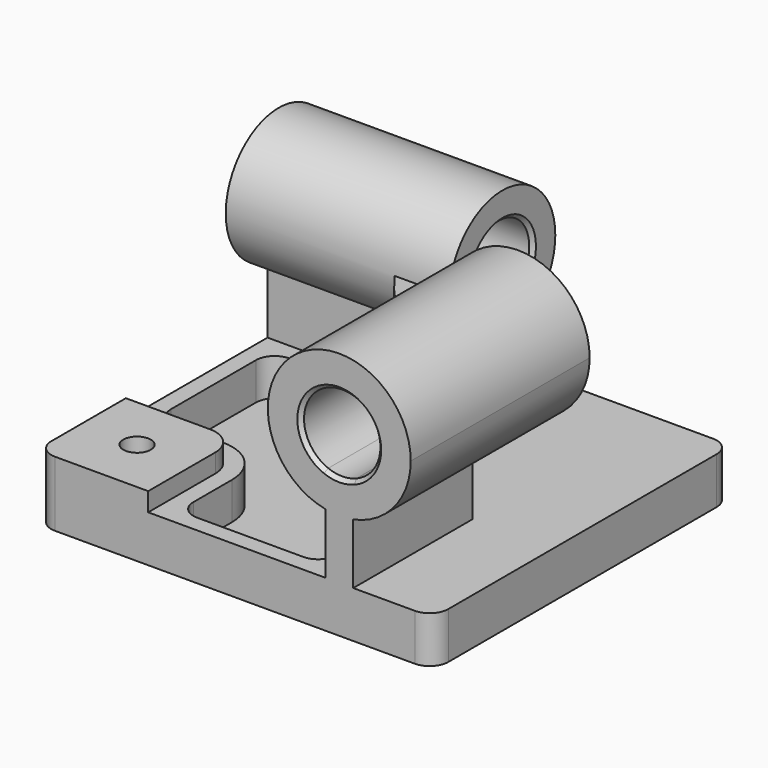
from build123d import *

# Parameters (mm, degrees)
F1_DEPTH       = 35
F2_DEPTH       = 25
F3_DEPTH       = 5
F4_DEPTH       = 95
F5_D           = 14.75
F5_CBORE_D     = 22.25
F5_CBORE_DEPTH = 14
F6_DEPTH       = 25
F8_DEPTH       = 120
F9_DEPTH       = 120
F11_DEPTH      = 120
F12_DEPTH      = 120
F13_SIZE       = 2


with BuildPart() as f1:
    # F0 (on Top) → F1 (new body)
    with BuildSketch(Plane.XY):
        with BuildLine():
            ThreePointArc((-106.5, 10), (-103.5710678119, 2.9289321881), (-96.5, 0))
            Line((-96.5, 0), (-46.5, 0))
            Line((-46.5, 0), (-46.5, 45))
            ThreePointArc((-46.5, 45), (-50.8933982822, 55.6066017178), (-61.5, 60))
            Line((-61.5, 60), (-106.5, 60))
            Line((-106.5, 60), (-106.5, 10))
        make_face()
    extrude(amount=F1_DEPTH)

    # F0 (on Top) → F2 (join)
    with BuildSketch(Plane.XY):
        with BuildLine():
            Line((-46.5, 45), (-46.5, 0))
            Line((-46.5, 0), (48.5, 0))
            Line((48.5, 0), (48.5, 9))
            Line((48.5, 9), (48.5, 73.0645805597))
            ThreePointArc((48.5, 73.0645805597), (0.9989947663, 106.8341893096), (-31.8154327598, 155))
            Line((-31.8154327598, 155), (-106.5, 155))
            Line((-106.5, 155), (-106.5, 60))
            Line((-106.5, 60), (-61.5, 60))
            ThreePointArc((-61.5, 60), (-50.8933982822, 55.6066017178), (-46.5, 45))
        make_face()
        with BuildLine():
            Line((-61.5, 69), (-87.5, 69))
            ThreePointArc((-87.5, 69), (-94.5710678119, 71.9289321881), (-97.5, 79))
            Line((-97.5, 79), (-97.5, 136))
            ThreePointArc((-97.5, 136), (-94.5710678119, 143.0710678119), (-87.5, 146))
            Line((-87.5, 146), (-44.0372922197, 146))
            ThreePointArc((-44.0372922197, 146), (-38.8802046252, 144.5676395548), (-35.2004786871, 140.6808895084))
            ThreePointArc((-35.2004786871, 140.6808895084), (-5.5795172138, 100.1842682312), (34.3477319863, 69.8001858066))
            ThreePointArc((34.3477319863, 69.8001858066), (38.1161859272, 66.1293498865), (39.5, 61.0537868568))
            Line((39.5, 61.0537868568), (39.5, 19))
            ThreePointArc((39.5, 19), (36.5710678119, 11.9289321881), (29.5, 9))
            Line((29.5, 9), (-27.5, 9))
            ThreePointArc((-27.5, 9), (-34.5710678119, 11.9289321881), (-37.5, 19))
            Line((-37.5, 19), (-37.5, 45))
            ThreePointArc((-37.5, 45), (-44.5294372515, 61.9705627485), (-61.5, 69))
        make_face(mode=Mode.SUBTRACT)
    extrude(amount=F2_DEPTH)

    # F0 (on Top) → F3 (join)
    with BuildSketch(Plane.XY):
        with BuildLine():
            ThreePointArc((-97.5, 79), (-94.5710678119, 71.9289321881), (-87.5, 69))
            Line((-87.5, 69), (-61.5, 69))
            ThreePointArc((-61.5, 69), (-44.5294372515, 61.9705627485), (-37.5, 45))
            Line((-37.5, 45), (-37.5, 19))
            ThreePointArc((-37.5, 19), (-34.5710678119, 11.9289321881), (-27.5, 9))
            Line((-27.5, 9), (29.5, 9))
            ThreePointArc((29.5, 9), (36.5710678119, 11.9289321881), (39.5, 19))
            Line((39.5, 19), (39.5, 61.0537868568))
            ThreePointArc((39.5, 61.0537868568), (38.1161859272, 66.1293498865), (34.3477319863, 69.8001858066))
            ThreePointArc((34.3477319863, 69.8001858066), (-5.5795172138, 100.1842682312), (-35.2004786871, 140.6808895084))
            ThreePointArc((-35.2004786871, 140.6808895084), (-38.8802046252, 144.5676395548), (-44.0372922197, 146))
            Line((-44.0372922197, 146), (-87.5, 146))
            ThreePointArc((-87.5, 146), (-94.5710678119, 143.0710678119), (-97.5, 136))
            Line((-97.5, 136), (-97.5, 79))
        make_face()
    extrude(amount=F3_DEPTH)

    # F0 (on Top) → F4 (join)
    with BuildSketch(Plane.XY):
        with BuildLine():
            Line((48.5, 9), (48.5, 0))
            Line((48.5, 0), (63.5, 0))
            Line((63.5, 0), (63.5, 80))
            ThreePointArc((63.5, 80), (11.2368967619, 117.7368967619), (-26.5, 170))
            Line((-26.5, 170), (-106.5, 170))
            Line((-106.5, 170), (-106.5, 155))
            Line((-106.5, 155), (-31.8154327598, 155))
            ThreePointArc((-31.8154327598, 155), (0.9989947663, 106.8341893096), (48.5, 73.0645805597))
            Line((48.5, 73.0645805597), (48.5, 9))
        make_face()
    extrude(amount=F4_DEPTH)

    # F5 (through all)
    with Locations(Plane(origin=(0, 0, 0), x_dir=(1, 0, 0), z_dir=(0, 0, -1))):
        with Locations((-76.5, -30)):
            CounterBoreHole(F5_D / 2, F5_CBORE_D / 2, F5_CBORE_DEPTH)

    # F0 (on Top) → F6 (join)
    with BuildSketch(Plane.XY):
        with BuildLine():
            Line((63.5, 80), (63.5, 0))
            Line((63.5, 0), (96.5, 0))
            ThreePointArc((96.5, 0), (103.5710678119, 2.9289321881), (106.5, 10))
            Line((106.5, 10), (106.5, 190))
            ThreePointArc((106.5, 190), (103.5710678119, 197.0710678119), (96.5, 200))
            Line((96.5, 200), (-96.5, 200))
            ThreePointArc((-96.5, 200), (-103.5710678119, 197.0710678119), (-106.5, 190))
            Line((-106.5, 190), (-106.5, 170))
            Line((-106.5, 170), (-26.5, 170))
            ThreePointArc((-26.5, 170), (11.2368967619, 117.7368967619), (63.5, 80))
        make_face()
    extrude(amount=F6_DEPTH)

    # F7 (on face) → F8 (cut)
    with BuildSketch(Plane.XZ):
        with BuildLine():
            Line((48.5, 75.9212159717), (48.5, 95))
            Line((48.5, 95), (63.5, 95))
            Line((63.5, 95), (63.5, 75.9212159717))
            ThreePointArc((63.5, 75.9212159717), (72.9410743461, 83.4566036194), (76.5, 95))
            ThreePointArc((76.5, 95), (44.4566036194, 111.9410743461), (48.5, 75.9212159717))
        make_face()
        with BuildLine():
            Line((63.5, 95), (48.5, 95))
            Line((48.5, 95), (48.5, 75.9212159717))
            ThreePointArc((48.5, 75.9212159717), (56, 74.5), (63.5, 75.9212159717))
            Line((63.5, 75.9212159717), (63.5, 95))
        make_face()
    extrude(amount=-F8_DEPTH, mode=Mode.SUBTRACT)

    # F7 (on face) → F9 (join)
    with BuildSketch(Plane.XZ):
        with BuildLine():
            Line((48.5, 57.4075197384), (48.5, 75.9212159717))
            ThreePointArc((48.5, 75.9212159717), (44.4566036194, 111.9410743461), (76.5, 95))
            ThreePointArc((76.5, 95), (72.9410743461, 83.4566036194), (63.5, 75.9212159717))
            Line((63.5, 75.9212159717), (63.5, 57.4075197384))
            ThreePointArc((63.5, 57.4075197384), (85.6390332562, 70.6900785715), (94.333335, 95))
            ThreePointArc((94.333335, 95), (31.6900785715, 124.6390332562), (48.5, 57.4075197384))
        make_face()
        with BuildLine():
            ThreePointArc((63.5, 75.9212159717), (56, 74.5), (48.5, 75.9212159717))
            Line((48.5, 75.9212159717), (48.5, 57.4075197384))
            ThreePointArc((48.5, 57.4075197384), (56, 56.666665), (63.5, 57.4075197384))
            Line((63.5, 57.4075197384), (63.5, 75.9212159717))
        make_face()
    extrude(amount=-F9_DEPTH)

    # F10 (on face) → F11 (cut)
    with BuildSketch(Plane(origin=(-106.5, 0, 0), x_dir=(0, -1, 0), z_dir=(-1, 0, 0))):
        with BuildLine():
            Line((-170, 95), (-155, 95))
            Line((-155, 95), (-155, 75.9212159717))
            ThreePointArc((-155, 75.9212159717), (-145.5589256539, 83.4566036194), (-142, 95))
            ThreePointArc((-142, 95), (-174.0433963806, 111.9410743461), (-170, 75.9212159717))
            Line((-170, 75.9212159717), (-170, 95))
        make_face()
        with BuildLine():
            Line((-155, 75.9212159717), (-155, 95))
            Line((-155, 95), (-170, 95))
            Line((-170, 95), (-170, 75.9212159717))
            ThreePointArc((-170, 75.9212159717), (-162.5, 74.5), (-155, 75.9212159717))
        make_face()
    extrude(amount=-F11_DEPTH, mode=Mode.SUBTRACT)

    # F10 (on face) → F12 (join)
    with BuildSketch(Plane(origin=(-106.5, 0, 0), x_dir=(0, -1, 0), z_dir=(-1, 0, 0))):
        with BuildLine():
            ThreePointArc((-142, 95), (-145.5589256539, 83.4566036194), (-155, 75.9212159717))
            Line((-155, 75.9212159717), (-155, 60.3012968542))
            ThreePointArc((-155, 60.3012968542), (-134.8730204329, 72.7065031904), (-127, 95))
            ThreePointArc((-127, 95), (-184.7934968096, 122.6269795671), (-170, 60.3012968542))
            Line((-170, 60.3012968542), (-170, 75.9212159717))
            ThreePointArc((-170, 75.9212159717), (-174.0433963806, 111.9410743461), (-142, 95))
        make_face()
        with BuildLine():
            Line((-155, 60.3012968542), (-155, 75.9212159717))
            ThreePointArc((-155, 75.9212159717), (-162.5, 74.5), (-170, 75.9212159717))
            Line((-170, 75.9212159717), (-170, 60.3012968542))
            ThreePointArc((-170, 60.3012968542), (-162.5, 59.5), (-155, 60.3012968542))
        make_face()
    extrude(amount=-F12_DEPTH)

    # F13
    f13_edges = [f1.edges().sort_by_distance(p)[0] for p in [
        (35.5, 0, 95),
        (35.5, 120, 95),
        (13.5, 183, 95),
        (-106.5, 162.5, 74.5),
        (-106.5, 145.558926, 83.456604),
        (-106.5, 174.043396, 111.941074),
    ]]
    chamfer(f13_edges, length=F13_SIZE)


solid = f1.part
